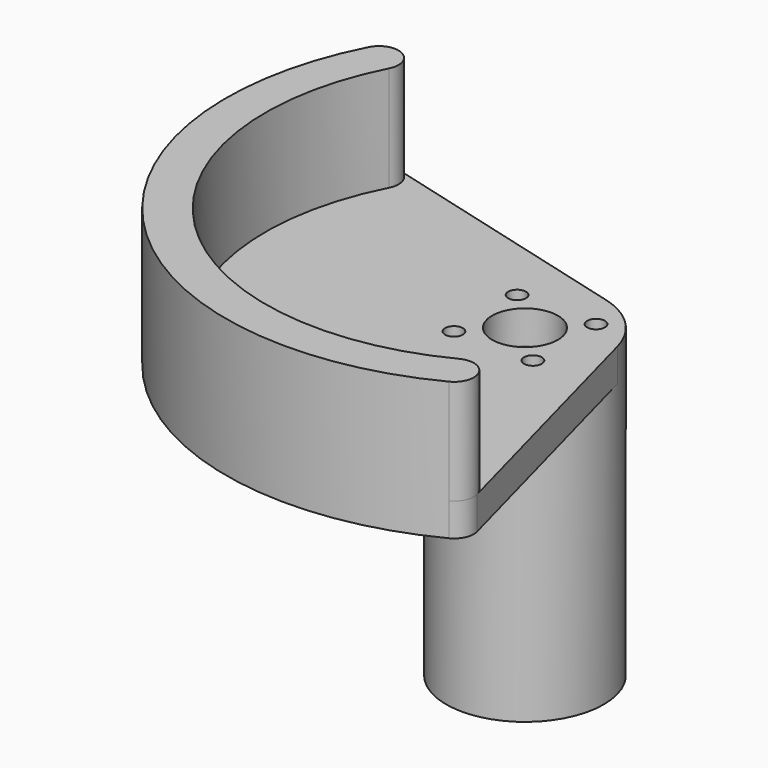
from build123d import *
from build123d import SkipClean  # not in build123d's __all__

# Parameters (mm, degrees)
F0_R     = 19.05
F0_R_2   = 2.15265
F1_DEPTH = 66.04
F3_DEPTH = 66.04
F4_COUNT = 4
F4_ANGLE = 270
F5_R     = 2.15265
F5_R_2   = 7.9375
F6_DEPTH = 7.9375
F8_DEPTH = 25.4


# Not quite as in the source:
# - after a boolean that leaves OpenCascade's solid faulty, fix() repairs it


with BuildPart() as f1:
    # F0 (on Top) → F1 (new body)
    with BuildSketch(Plane.XY):
        Circle(F0_R)
        with Locations((-9.5415221286, -9.5415221286)):
            Circle(F0_R_2, mode=Mode.SUBTRACT)
        with Locations((9.5415221286, -9.5415221286)):
            Circle(F0_R_2, mode=Mode.SUBTRACT)
        with Locations((-9.5415221286, 9.5415221286)):
            Circle(F0_R_2, mode=Mode.SUBTRACT)
        with BuildLine():
            ThreePointArc((0, 7.9375), (5.6126600757, 5.6126600757), (7.9375, 0))
            ThreePointArc((7.9375, 0), (-5.6126600757, -5.6126600757), (0, 7.9375))
        make_face(mode=Mode.SUBTRACT)
        with Locations((9.5415221286, 9.5415221286)):
            Circle(F0_R_2, mode=Mode.SUBTRACT)
    extrude(amount=F1_DEPTH)

    # F2 (on face) → F3 (cut, through all)
    with BuildSketch(Plane(origin=(0, 0, 0), x_dir=(1, 0, 0), z_dir=(0, 0, -1))):
        with BuildLine():
            ThreePointArc((8.8488960712, -15.0544327217), (5.6543471209, -13.5116335278), (4.0444600337, -10.350362278))
            ThreePointArc((4.0444600337, -10.350362278), (0, -11.1125), (-4.0444600337, -10.350362278))
            ThreePointArc((-4.0444600337, -10.350362278), (-5.6543471209, -13.5116335278), (-8.8488960712, -15.0544327217))
            ThreePointArc((-8.8488960712, -15.0544327217), (0, -17.4625), (8.8488960712, -15.0544327217))
        make_face()
    f3 = extrude(amount=-F3_DEPTH, mode=Mode.SUBTRACT)

    # F4: F3 ×4 about axis
    f4_axis = Axis((0, 0, 0), (0, 0, -1))
    for i in range(1, F4_COUNT):
        add(f3.rotate(f4_axis, i * F4_ANGLE / (F4_COUNT - 1)), clean=False, mode=Mode.SUBTRACT)

    # F5 (on face) → F6 (join)
    with BuildSketch(Plane.XY.offset(66.04)):
        with BuildLine():
            Line((35.4737477046, -58.7862808051), (18.4008869908, 4.9305028092))
            ThreePointArc((18.4008869908, 4.9305028092), (13.4703841816, 13.4703841816), (4.9305028092, 18.4008869908))
            Line((4.9305028092, 18.4008869908), (-58.7862808051, 35.4737477046))
            ThreePointArc((-58.7862808051, 35.4737477046), (-61.9475900585, 35.228016284), (-64.2539485249, 33.05201749))
            ThreePointArc((-64.2539485249, 33.05201749), (-51.093080555, -51.093080555), (33.05201749, -64.2539485249))
            ThreePointArc((33.05201749, -64.2539485249), (35.228016284, -61.9475900585), (35.4737477046, -58.7862808051))
        make_face()
        with Locations((-9.5415221286, -9.5415221286)):
            Circle(F5_R, mode=Mode.SUBTRACT)
        Circle(F5_R_2, mode=Mode.SUBTRACT)
        with Locations((9.5415221286, -9.5415221286)):
            Circle(F5_R, mode=Mode.SUBTRACT)
        with Locations((-9.5415221286, 9.5415221286)):
            Circle(F5_R, mode=Mode.SUBTRACT)
        with Locations((9.5415221286, 9.5415221286)):
            Circle(F5_R, mode=Mode.SUBTRACT)
    with SkipClean():  # cleaning this boolean's faces spoils the solid; the shape is the same uncleaned
        extrude(amount=F6_DEPTH)

    # F7 (on face) → F8 (join)
    with BuildSketch(Plane.XY.offset(73.9775)):
        with BuildLine():
            ThreePointArc((-55.7838644899, 28.6950344237), (-57.8404149742, 35.1085679744), (-64.2539485249, 33.05201749))
            ThreePointArc((-64.2539485249, 33.05201749), (-51.093080555, -51.093080555), (33.05201749, -64.2539485249))
            ThreePointArc((33.05201749, -64.2539485249), (35.1085679744, -57.8404149742), (28.6950344237, -55.7838644899))
            ThreePointArc((28.6950344237, -55.7838644899), (-44.3578884642, -44.3578884642), (-55.7838644899, 28.6950344237))
        make_face()
    extrude(amount=F8_DEPTH)

    add(f1.part.fix(), mode=Mode.REPLACE)


solid = f1.part
